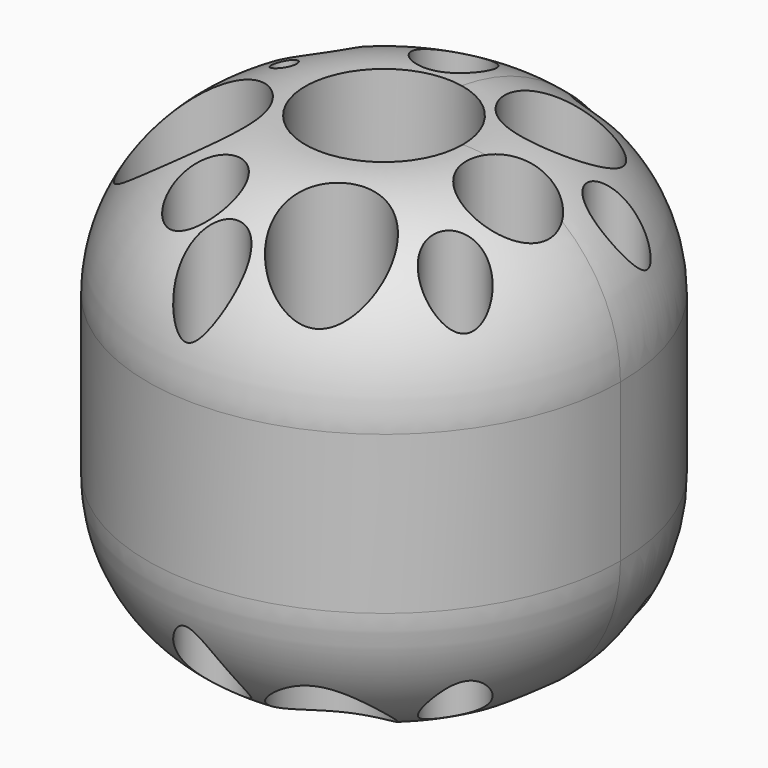
from build123d import *

# Parameters (mm, degrees)
F0_R        = 38.1
F1_DEPTH    = 76.2
F2_R        = 12.7
F3_DEPTH    = 180.848
F4_R        = 7.051388811
F4_R_2      = 10.0077567436
F4_R_3      = 8.3643094525
F4_R_4      = 5.4559046701
F4_R_5      = 8.2156500919
F4_R_6      = 6.9156415044
F4_R_7      = 4.7098788649
F4_R_8      = 6.1115303
F4_R_9      = 5.6605710863
F4_R_10     = 4.4882950914
F4_R_11     = 3.4721806932
F4_R_12     = 1.8443699081
F4_R_13     = 4.2964234472
F4_R_14     = 3.6887398162
F4_R_15     = 4.9256604094
F5_DEPTH    = 128.27
F6_T2_ANGLE = 281.6017699754
F6_T4_ANGLE = 266.0855324395
F7_T2_ANGLE = 281.6017699754
F7_T4_ANGLE = 266.0855324395


# Not quite as in the source:
# - a fillet or chamfer that OpenCascade refuses, or shapes differently, is made with other operations: its cross-section is extruded or revolved along the edge and cut away or added


with BuildPart() as f1:
    # F0 (on Top) → F1 (new body)
    with BuildSketch(Plane.XY):
        Circle(F0_R)
    extrude(amount=-F1_DEPTH)

    # F2 (on face) → F3 (cut)
    with BuildSketch(Plane(origin=(0, 0, -76.2), x_dir=(1, 0, 0), z_dir=(0, 0, -1))):
        Circle(F2_R)
    extrude(amount=-F3_DEPTH, mode=Mode.SUBTRACT)

    # F4 (on Top) → F5 (cut)
    with BuildSketch(Plane.XY):
        with Locations((-23.8397140056, 15.5665706843)):
            Circle(F4_R)
        with Locations((-22.0980010927, -10.7768569142)):
            Circle(F4_R_2)
        with Locations((10.7768569142, -24.0574292839)):
            Circle(F4_R_3)
        with Locations((-9.6882851794, -23.8397140056)):
            Circle(F4_R_4)
        with Locations((16.2197146565, 15.3488572687)):
            Circle(F4_R_5)
        with Locations((22.5334297866, -3.1568570994)):
            Circle(F4_R_6)
        with Locations((25.1460019499, -17.0905720443)):
            Circle(F4_R_7)
        with Locations((-14.260285534, 27.7585722506)):
            Circle(F4_R_8)
        with Locations((-4.0277135558, 19.0500002354)):
            Circle(F4_R_9)
        with Locations((2.9391427524, 32.5482860208)):
            Circle(F4_R_10)
        with Locations((-34.5041453838, 4.6927542426)):
            Circle(F4_R_11)
        with Locations((-20.1897285879, 5.140079651)):
            Circle(F4_R_12)
        with Locations((30.1343873143, 9.1660087928)):
            Circle(F4_R_13)
        with Locations((11.3467173651, 29.2956568301)):
            Circle(F4_R_14)
        with Locations((-2.0730462857, -31.9879353046)):
            Circle(F4_R_15)
    extrude(amount=-F5_DEPTH, mode=Mode.SUBTRACT)

    # F6: fillet of radius 25.4 on 1 edges, made by hand

    # F6_s1 → F6_t2 (revolve, cut)
    with BuildSketch(Plane(origin=(0, 0, 0), x_dir=(0, 0, 1), z_dir=(0.9795690375, -0.201108182, 0))):
        with BuildLine():
            ThreePointArc((-76.2, -12.7), (-68.7605122421, -30.6605122421), (-50.8, -38.1))
            Line((-50.8, -38.1), (-76.2, -38.1))
            Line((-76.2, -38.1), (-76.2, -12.7))
        make_face()
    revolve(axis=Axis((0, 0, -76.2), (0, 0, 1)), revolution_arc=F6_T2_ANGLE, mode=Mode.SUBTRACT)

    # F6_s3 → F6_t4 (revolve, cut)
    with BuildSketch(Plane.XZ):
        with BuildLine():
            ThreePointArc((38.1, -50.8), (30.6605122421, -68.7605122421), (12.7, -76.2))
            Line((12.7, -76.2), (38.1, -76.2))
            Line((38.1, -76.2), (38.1, -50.8))
        make_face()
    revolve(axis=Axis((0, 0, -76.2), (0, 0, 1)), revolution_arc=F6_T4_ANGLE, mode=Mode.SUBTRACT)

    # F7: fillet of radius 25.4 on 1 edges, made by hand

    # F7_s1 → F7_t2 (revolve, cut)
    with BuildSketch(Plane(origin=(0, 0, 0), x_dir=(0, 0, 1), z_dir=(0.9795690375, -0.201108182, 0))):
        with BuildLine():
            ThreePointArc((-25.4, -38.1), (-7.4394877579, -30.6605122421), (0, -12.7))
            Line((0, -12.7), (0, -38.1))
            Line((0, -38.1), (-25.4, -38.1))
        make_face()
    revolve(axis=Axis((0, 0, 0), (0, 0, 1)), revolution_arc=F7_T2_ANGLE, mode=Mode.SUBTRACT)

    # F7_s3 → F7_t4 (revolve, cut)
    with BuildSketch(Plane.XZ):
        with BuildLine():
            ThreePointArc((38.1, -25.4), (30.6605122421, -7.4394877579), (12.7, 0))
            Line((12.7, 0), (38.1, 0))
            Line((38.1, 0), (38.1, -25.4))
        make_face()
    revolve(axis=Axis((0, 0, 0), (0, 0, 1)), revolution_arc=F7_T4_ANGLE, mode=Mode.SUBTRACT)


solid = f1.part
